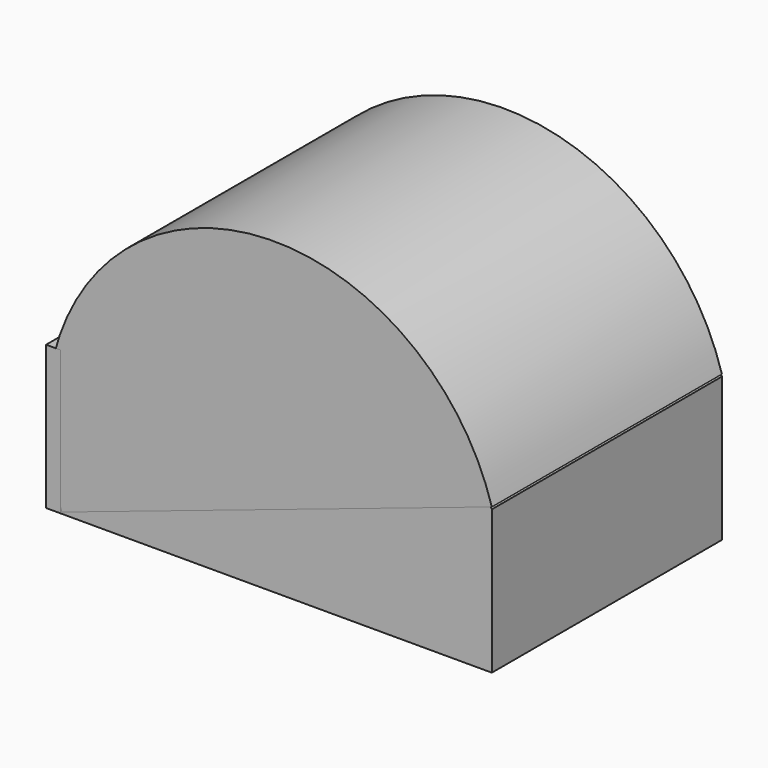
from build123d import *

# Parameters (mm, degrees)
F0_W     = 60
F0_H     = 20
F1_DEPTH = 40
F3_DEPTH = 40
F4_W     = 40
F4_H     = 20
F5_DEPTH = 2


# Not quite as in the source:
# - a feature names something its author has since deleted; it is built from what else it names


with BuildPart() as f1:
    # F0 (on Front) → F1 (new body)
    with BuildSketch(Plane.XZ):
        with Locations((-2.7382690459, -23.8184666568)):
            Rectangle(F0_W, F0_H)
        with BuildLine():
            ThreePointArc((27.2617309541, -13.8184666568), (-2.7382690459, 5.032068405), (-32.7382690459, -13.8184666568))
            Line((-32.7382690459, -13.8184666568), (27.2617309541, -13.8184666568))
        make_face()
    extrude(amount=F1_DEPTH)


with BuildPart() as f3:
    # F2 (on Front) → F3 (new body)
    with BuildSketch(Plane.XZ):
        with BuildLine():
            Line((-32.5370542705, -33.5944630206), (27.2599291056, -13.5201252997))
            ThreePointArc((27.2599291056, -13.5201252997), (-13.0723634113, 7.5226758687), (-32.5370542705, -33.5944630206))
        make_face()
    extrude(amount=F3_DEPTH)


with BuildPart() as f5:
    # F4 (on face) → F5 (new body)
    with BuildSketch(Plane(origin=(-32.7382690459, 0, 0), x_dir=(0, -1, 0), z_dir=(-1, 0, 0))):
        with Locations((20, -23.8184666568)):
            Rectangle(F4_W, F4_H)
    extrude(amount=F5_DEPTH)


solid = Compound([f1.part, f3.part, f5.part])
